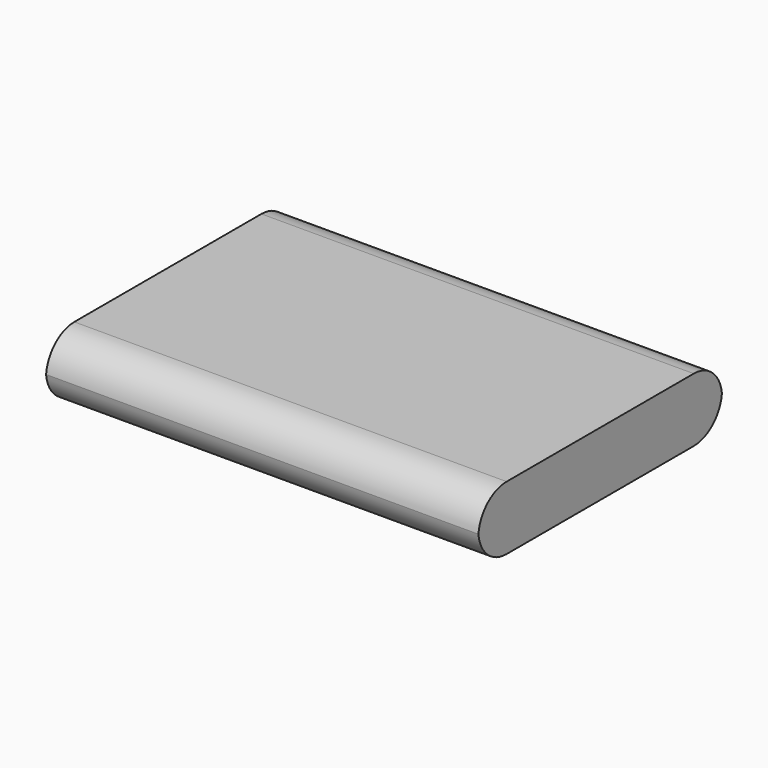
from build123d import *

# Parameters (mm, degrees)
F0_W        = 61
F0_H        = 43
F1_DEPTH    = 9
F2_T1_DEPTH = 86


# Not quite as in the source:
# - a fillet or chamfer that OpenCascade refuses, or shapes differently, is made with other operations: its cross-section is extruded or revolved along the edge and cut away or added


with BuildPart() as f1:
    # F0 (on Top) → F1 (new body)
    with BuildSketch(Plane.XY):
        Rectangle(F0_W, F0_H)
    extrude(amount=F1_DEPTH)

    # F2: fillet of radius 5 on 4 edges, made by hand

    # F2_s2 → F2_t1 (cut)
    with BuildSketch(Plane.YZ.offset(-43)):
        with BuildLine():
            ThreePointArc((21.5, 4), (20.0355339059, 7.5355339059), (16.5, 9))
            Line((16.5, 9), (21.5, 9))
            Line((21.5, 9), (21.5, 4))
        make_face()
        with BuildLine():
            ThreePointArc((-21.5, 4), (-20.0355339059, 7.5355339059), (-16.5, 9))
            Line((-16.5, 9), (-21.5, 9))
            Line((-21.5, 9), (-21.5, 4))
        make_face()
        with BuildLine():
            ThreePointArc((-21.5, 5), (-20.0355339059, 1.4644660941), (-16.5, 0))
            Line((-16.5, 0), (-21.5, 0))
            Line((-21.5, 0), (-21.5, 5))
        make_face()
        with BuildLine():
            ThreePointArc((21.5, 5), (20.0355339059, 1.4644660941), (16.5, 0))
            Line((16.5, 0), (21.5, 0))
            Line((21.5, 0), (21.5, 5))
        make_face()
    extrude(amount=F2_T1_DEPTH, mode=Mode.SUBTRACT)


solid = f1.part
